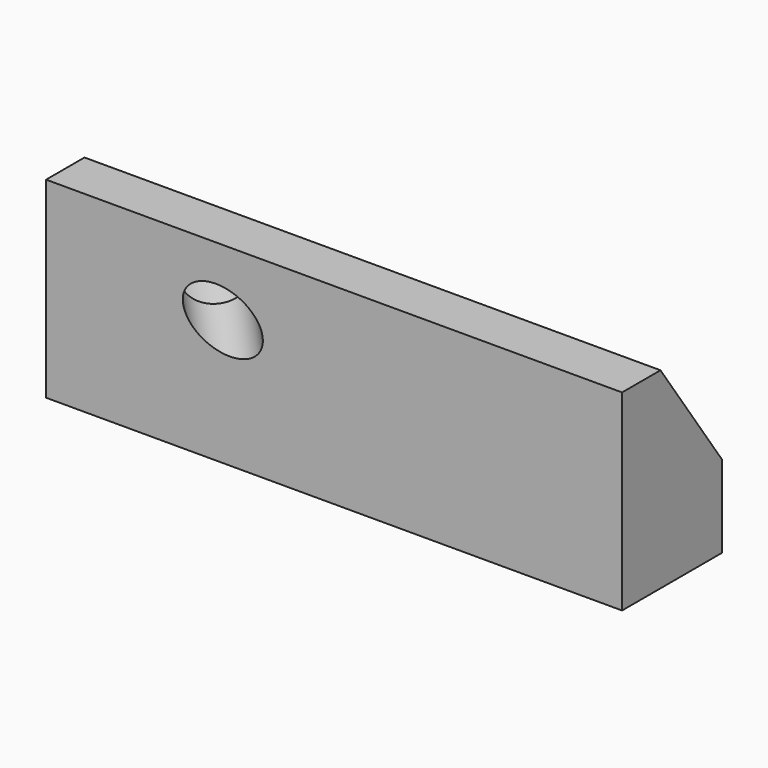
from build123d import *

# Parameters (mm, degrees)
F0_W      = 30
F0_H      = 10
F1_DEPTH  = 6.5
F6_SIZE2  = 5.712592027
F6_SIZE   = 4
F9_R      = 1.5
F10_DEPTH = 12.5
F12_R     = 2.5
F13_DEPTH = 22


with BuildPart() as f1:
    # F0 (on Front) → F1 (new body)
    with BuildSketch(Plane.XZ):
        Rectangle(F0_W, F0_H)
    extrude(amount=F1_DEPTH)

    # F6
    f6_edges = [f1.edges().sort_by_distance(p)[0] for p in [
        (0, 0, 5),
    ]]
    f6_side = f1.faces().sort_by_distance((0, -3.25, 5))[0]
    chamfer(f6_edges, length=F6_SIZE, length2=F6_SIZE2, reference=f6_side)

    # F9 (on face) → F10 (cut, symmetric)
    with BuildSketch(Plane(origin=(0.2414814566, -0.25, -0.0647047613), x_dir=(-0.7304064958, -0.6612248329, -0.1711375799), z_dir=(-0.6830127019, 0.7071067812, 0.1830127019))):
        with Locations((8.2653104118, 3.1320350886)):
            Circle(F9_R)
    extrude(amount=F10_DEPTH, both=True, mode=Mode.SUBTRACT)

    # F12 (on face) → F13 (cut)
    with BuildSketch(Plane(origin=(-16.8338360907, 17.4276695297, 4.510612786), x_dir=(-0.7304064958, -0.6612248329, -0.1711375799), z_dir=(-0.6830127019, 0.7071067812, 0.1830127019))):
        with Locations((8.2653104118, 3.1320350886)):
            Circle(F12_R)
    extrude(amount=-F13_DEPTH, mode=Mode.SUBTRACT)


solid = f1.part
